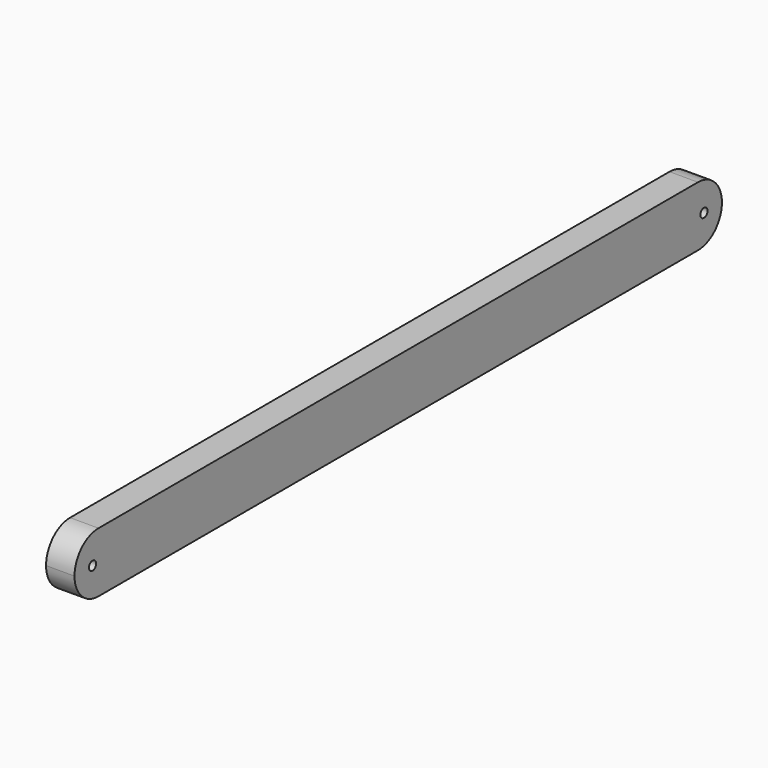
from build123d import *

# Parameters (mm, degrees)
F0_W     = 540
F0_H     = 40
F0_R     = 3
F1_DEPTH = 19
F2_R     = 19.99999


# Not quite as in the source:
# - a fillet or chamfer is up to 0.001 mm smaller than in the source, because OpenCascade refuses the exact size


with BuildPart() as f1:
    # F0 (on Right) → F1 (new body)
    with BuildSketch(Plane.YZ):
        with Locations((-255, 0)):
            Rectangle(F0_W, F0_H)
        with Locations((-510, 0)):
            Circle(F0_R, mode=Mode.SUBTRACT)
        Circle(F0_R, mode=Mode.SUBTRACT)
    extrude(amount=F1_DEPTH)

    # F2 (radius 20 in the source; OpenCascade refuses exactly that, so slightly less here)
    f2_edges = [f1.edges().sort_by_distance(p)[0] for p in [
        (9.5, 15, 20),
        (9.5, 15, -20),
        (9.5, -525, 20),
        (9.5, -525, -20),
    ]]
    fillet(f2_edges, radius=F2_R)


solid = f1.part
